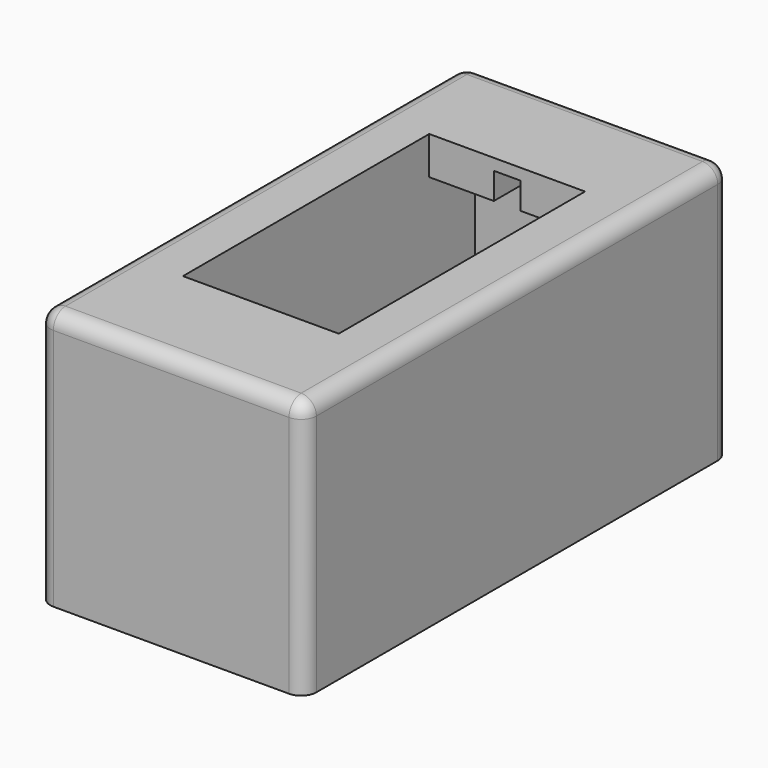
from build123d import *

# Parameters (mm, degrees)
F0_W      = 35
F0_H      = 70
F1_DEPTH  = 40
F2_W      = 20.5
F2_H      = 55.6
F3_DEPTH  = 35
F4_W      = 20.5
F4_H      = 40.5
F5_DEPTH  = 25
F6_DEPTH  = 6
F7_W      = 3.5
F7_H      = 6
F8_DEPTH  = 3.5
F10_D     = 4.2
F10_DEPTH = 15
F10_TIP   = 1.2618073
F11_R     = 2
F12_W     = 9
F12_H     = 6
F13_DEPTH = 10


# Not quite as in the source:
# - a pattern or mirror of a feature is missing from the dataset's text; its kind, count and spacing are read off the source's solid


with BuildPart() as f1:
    # F0 (on Top) → F1 (new body)
    with BuildSketch(Plane.XY):
        Rectangle(F0_W, F0_H)
    extrude(amount=F1_DEPTH)

    # F2 (on face) → F3 (cut)
    with BuildSketch(Plane(origin=(0, 0, 0), x_dir=(1, 0, 0), z_dir=(0, 0, -1))):
        Rectangle(F2_W, F2_H)
    extrude(amount=-F3_DEPTH, mode=Mode.SUBTRACT)

    # F4 (on face) → F5 (cut)
    with BuildSketch(Plane.XY.offset(40)):
        Rectangle(F4_W, F4_H)
    extrude(amount=-F5_DEPTH, mode=Mode.SUBTRACT)

    # F6 (cut): a face of the model
    f6_faces = [f1.faces().sort_by_distance(p)[0] for p in [
        (16.7173762079, 0, 0),
    ]]
    extrude(f6_faces, amount=-F6_DEPTH, mode=Mode.SUBTRACT)

    # F7 (on face) → F8 (cut)
    with BuildSketch(Plane(origin=(0, 0, 35), x_dir=(1, 0, 0), z_dir=(0, 0, -1))):
        with Locations((0, 23.25)):
            Rectangle(F7_W, F7_H)
    f8 = extrude(amount=-F8_DEPTH, mode=Mode.SUBTRACT)

    # F8_copies: F8 across plane
    add(f8.mirror(Plane.ZX), mode=Mode.SUBTRACT)

    # F10
    with Locations(Plane(origin=(0, 0, 6), x_dir=(1, 0, 0), z_dir=(0, 0, -1))):
        with Locations((-13.875, 31.4), (13.875, 31.4), (13.875, -31.4), (-13.875, -31.4)):
            Hole(F10_D / 2, depth=F10_DEPTH)
            with Locations((0, 0, -(F10_DEPTH + F10_TIP / 2))):  # 118° drill point
                Cone(0, F10_D / 2, F10_TIP, mode=Mode.SUBTRACT)

    # F11
    f11_edges = [f1.edges().sort_by_distance(p)[0] for p in [
        (17.5, -35, 23),
        (17.5, 0, 40),
        (0, -35, 40),
        (-17.5, 0, 40),
        (17.5, 35, 23),
        (0, 35, 40),
        (-17.5, -35, 23),
        (-17.5, 35, 23),
    ]]
    fillet(f11_edges, radius=F11_R)

    # F12 (on face) → F13 (cut)
    with BuildSketch(Plane(origin=(0, 35, 0), x_dir=(-1, 0, 0), z_dir=(0, 1, 0))):
        with Locations((0, 9)):
            Rectangle(F12_W, F12_H)
    extrude(amount=-F13_DEPTH, mode=Mode.SUBTRACT)


solid = f1.part
